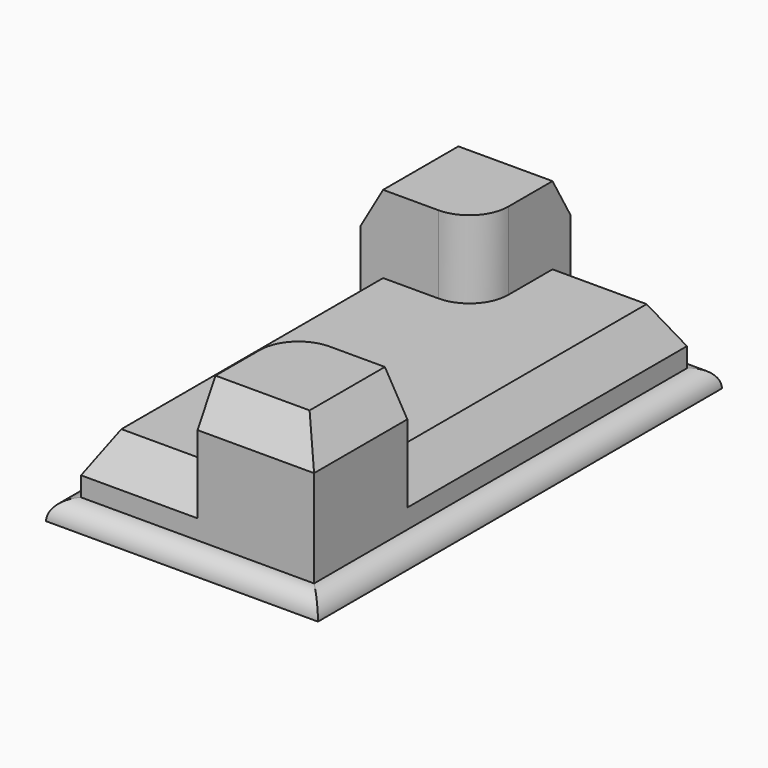
from build123d import *

# Parameters (mm, degrees)
F0_W     = 88.9
F0_H     = 165.1
F1_DEPTH = 6.35
F2_DEPTH = 25.4
F3_DEPTH = 50.8
F4_R     = 6.34999
F5_SIZE2 = 12.7
F5_SIZE  = 7.3323484187
F6_SIZE2 = 12.7
F6_SIZE  = 7.3323484187
F7_SIZE2 = 12.7
F7_SIZE  = 7.3323484187


# Not quite as in the source:
# - a fillet or chamfer is up to 0.001 mm smaller than in the source, because OpenCascade refuses the exact size


with BuildPart() as f1:
    # F0 (on Top) → F1 (new body)
    with BuildSketch(Plane.XY):
        with Locations((-38.1, 76.2)):
            Rectangle(F0_W, F0_H)
        Polygon((-76.2, 114.3), (-76.2, 152.4), (-38.1, 152.4), (0, 152.4), (0, 38.1), (0, 0), (-38.1, 0), (-76.2, 0), align=None, mode=Mode.SUBTRACT)
    extrude(amount=F1_DEPTH)

    # F0 (on Top) → F2 (join)
    with BuildSketch(Plane.XY):
        with BuildLine():
            Line((0, 152.4), (-38.1, 152.4))
            Line((-38.1, 152.4), (-38.1, 127))
            ThreePointArc((-38.1, 127), (-41.8197438789, 118.0197438789), (-50.8, 114.3))
            Line((-50.8, 114.3), (-76.2, 114.3))
            Line((-76.2, 114.3), (-76.2, 0))
            Line((-76.2, 0), (-38.1, 0))
            Line((-38.1, 0), (-38.1, 25.4))
            ThreePointArc((-38.1, 25.4), (-34.3802561211, 34.3802561211), (-25.4, 38.1))
            Line((-25.4, 38.1), (0, 38.1))
            Line((0, 38.1), (0, 152.4))
        make_face()
    extrude(amount=F2_DEPTH)

    # F0 (on Top) → F3 (join)
    with BuildSketch(Plane.XY):
        with BuildLine():
            Line((-38.1, 152.4), (-76.2, 152.4))
            Line((-76.2, 152.4), (-76.2, 114.3))
            Line((-76.2, 114.3), (-50.8, 114.3))
            ThreePointArc((-50.8, 114.3), (-41.8197438789, 118.0197438789), (-38.1, 127))
            Line((-38.1, 127), (-38.1, 152.4))
        make_face()
        with BuildLine():
            Line((0, 0), (0, 38.1))
            Line((0, 38.1), (-25.4, 38.1))
            ThreePointArc((-25.4, 38.1), (-34.3802561211, 34.3802561211), (-38.1, 25.4))
            Line((-38.1, 25.4), (-38.1, 0))
            Line((-38.1, 0), (0, 0))
        make_face()
    extrude(amount=F3_DEPTH)

    # F4 (radius 6.35 in the source; OpenCascade refuses exactly that, so slightly less here)
    f4_edges = [f1.edges().sort_by_distance(p)[0] for p in [
        (6.35, 76.2, 6.35),
        (-38.1, 158.75, 6.35),
        (-82.55, 76.2, 6.35),
        (-38.1, -6.35, 6.35),
    ]]
    fillet(f4_edges, radius=F4_R)

    # F5
    f5_edges = [f1.edges().sort_by_distance(p)[0] for p in [
        (0, 95.25, 25.4),
        (-57.15, 0, 25.4),
        (-76.2, 57.15, 25.4),
        (-19.05, 152.4, 25.4),
    ]]
    f5_side = f1.faces().sort_by_distance((-38.1, 76.2, 25.4))[0]
    chamfer(f5_edges, length=F5_SIZE, length2=F5_SIZE2, reference=f5_side)

    # F6
    f6_edges = [f1.edges().sort_by_distance(p)[0] for p in [
        (-57.15, 152.4, 50.8),
        (-76.2, 133.35, 50.8),
    ]]
    f6_side = f1.faces().sort_by_distance((-57.546042, 133.746042, 50.8))[0]
    chamfer(f6_edges, length=F6_SIZE, length2=F6_SIZE2, reference=f6_side)

    # F7
    f7_edges = [f1.edges().sort_by_distance(p)[0] for p in [
        (0, 19.05, 50.8),
        (-19.05, 0, 50.8),
    ]]
    f7_side = f1.faces().sort_by_distance((-18.653958, 18.653958, 50.8))[0]
    chamfer(f7_edges, length=F7_SIZE, length2=F7_SIZE2, reference=f7_side)


solid = f1.part
